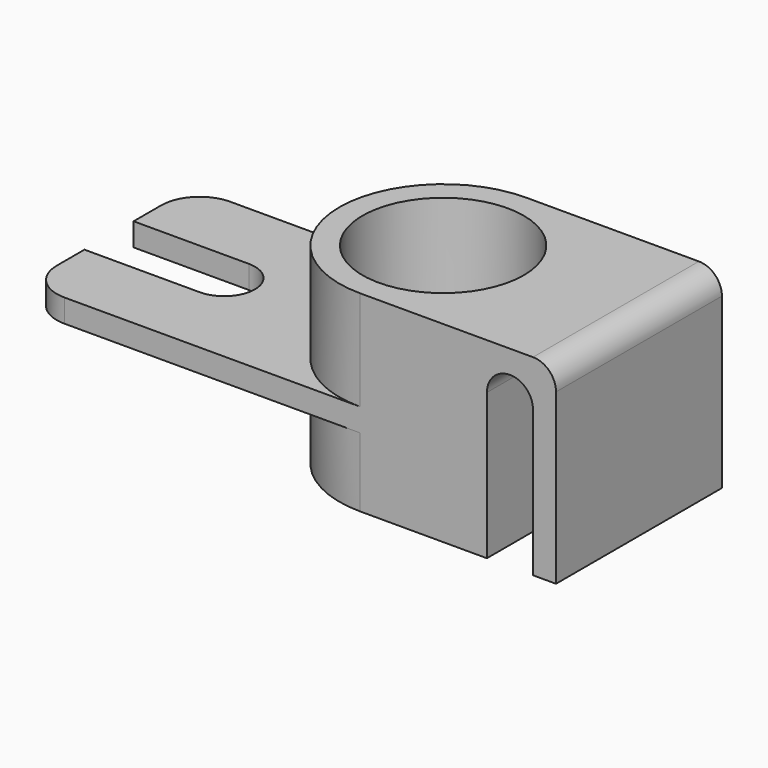
from build123d import *

# Parameters (mm, degrees)
F0_R     = 10.5
F0_W     = 6
F0_H     = 27
F0_W_2   = 3
F1_DEPTH = 3
F2_DEPTH = 22
F3_R     = 2.99999
F5_R     = 10.5
F6_DEPTH = 12
F7_DEPTH = 3
F8_R     = 5


# Not quite as in the source:
# - a fillet or chamfer is up to 0.001 mm smaller than in the source, because OpenCascade refuses the exact size


with BuildPart() as f1:
    # F0 (on Top) → F1 (new body)
    with BuildSketch(Plane.XY):
        with BuildLine():
            ThreePointArc((0, -13.5), (9.545941546, -9.545941546), (13.5, 0))
            ThreePointArc((13.5, 0), (9.545941546, 9.545941546), (0, 13.5))
            ThreePointArc((0, 13.5), (-13.5, 0), (0, -13.5))
        make_face()
        Circle(F0_R, mode=Mode.SUBTRACT)
        with BuildLine():
            Line((13.5, -13.5), (13.5, 0))
            ThreePointArc((13.5, 0), (9.545941546, -9.545941546), (0, -13.5))
            Line((0, -13.5), (13.5, -13.5))
        make_face()
        with BuildLine():
            ThreePointArc((0, 13.5), (9.545941546, 9.545941546), (13.5, 0))
            Line((13.5, 0), (13.5, 13.5))
            Line((13.5, 13.5), (0, 13.5))
        make_face()
        Polygon((13.5, 13.5), (13.5, 0), (13.5, -13.5), (16.5, -13.5), (16.5, 13.5), align=None)
        with Locations((19.5, 0)):
            Rectangle(F0_W, F0_H)
        with Locations((24, 0)):
            Rectangle(F0_W_2, F0_H)
    extrude(amount=F1_DEPTH)

    # F0 (on Top) → F2 (join)
    with BuildSketch(Plane.XY):
        with BuildLine():
            ThreePointArc((0, -13.5), (9.545941546, -9.545941546), (13.5, 0))
            ThreePointArc((13.5, 0), (9.545941546, 9.545941546), (0, 13.5))
            ThreePointArc((0, 13.5), (-13.5, 0), (0, -13.5))
        make_face()
        Circle(F0_R, mode=Mode.SUBTRACT)
        with BuildLine():
            ThreePointArc((0, 13.5), (9.545941546, 9.545941546), (13.5, 0))
            Line((13.5, 0), (13.5, 13.5))
            Line((13.5, 13.5), (0, 13.5))
        make_face()
        Polygon((13.5, 13.5), (13.5, 0), (13.5, -13.5), (16.5, -13.5), (16.5, 13.5), align=None)
        with Locations((24, 0)):
            Rectangle(F0_W_2, F0_H)
        with BuildLine():
            Line((13.5, -13.5), (13.5, 0))
            ThreePointArc((13.5, 0), (9.545941546, -9.545941546), (0, -13.5))
            Line((0, -13.5), (13.5, -13.5))
        make_face()
    extrude(amount=-F2_DEPTH)

    # F3 (radius 3 in the source; OpenCascade refuses exactly that, so slightly less here)
    f3_edges = [f1.edges().sort_by_distance(p)[0] for p in [
        (16.5, 0, 0),
        (22.5, 0, 0),
        (25.5, 0, 3),
    ]]
    fillet(f3_edges, radius=F3_R)



with BuildPart() as f6:
    # F5 (on offset) → F6 (new body)
    with BuildSketch(Plane(origin=(0, 0, -10), x_dir=(1, 0, 0), z_dir=(0, 0, -1))):
        with BuildLine():
            Line((16.5, 13.5), (0, 13.5))
            ThreePointArc((0, 13.5), (-13.5, 0), (0, -13.5))
            Line((0, -13.5), (16.5, -13.5))
            Line((16.5, -13.5), (16.5, 13.5))
        make_face()
        Circle(F5_R, mode=Mode.SUBTRACT)
    extrude(amount=-F6_DEPTH)


with BuildPart() as f1_1:
    add(f1.part)

    add(f6.part)  # F7 merges F6
    # F5 (on offset) → F7 (join)
    with BuildSketch(Plane(origin=(0, 0, -10), x_dir=(1, 0, 0), z_dir=(0, 0, -1))):
        with BuildLine():
            Line((16.5, 13.5), (0, 13.5))
            ThreePointArc((0, 13.5), (-13.5, 0), (0, -13.5))
            Line((0, -13.5), (16.5, -13.5))
            Line((16.5, -13.5), (16.5, 13.5))
        make_face()
        Circle(F5_R, mode=Mode.SUBTRACT)
        with BuildLine():
            ThreePointArc((0, -13.5), (-13.5, 0), (0, 13.5))
            Line((0, 13.5), (-43.5, 13.5))
            Line((-43.5, 13.5), (-43.5, 4))
            Line((-43.5, 4), (-28.5, 4))
            ThreePointArc((-28.5, 4), (-24.5, 0), (-28.5, -4))
            Line((-28.5, -4), (-43.5, -4))
            Line((-43.5, -4), (-43.5, -13.5))
            Line((-43.5, -13.5), (0, -13.5))
        make_face()
    extrude(amount=F7_DEPTH)

    # F8
    f8_edges = [f1_1.edges().sort_by_distance(p)[0] for p in [
        (-43.5, -13.5, -11.5),
        (-43.5, 13.5, -11.5),
    ]]
    fillet(f8_edges, radius=F8_R)


solid = f1_1.part
